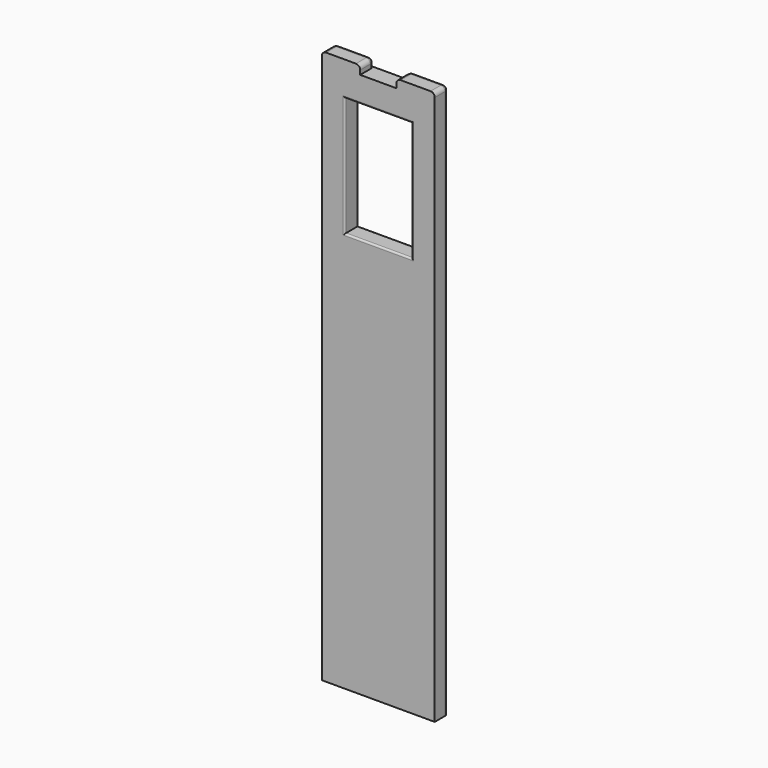
from build123d import *

# Parameters (mm, degrees)
F0_W     = 13.25
F0_H     = 65
F0_W_2   = 7.85
F0_H_2   = 14
F1_DEPTH = 2
F3_W     = 4.25
F3_H     = 2.1652186014
F4_DEPTH = 25
F5_R     = 0.5
F6_R     = 0.5
F7_R     = 0.2
F8_R     = 0.5


# Not quite as in the source:
# - the program builds the solid bodies; features that only make, move or delete a surface that nothing else refers to are left out


with BuildPart() as f1:
    # F0 (on Front) → F1 (new body)
    with BuildSketch(Plane.XZ):
        Rectangle(F0_W, F0_H)
        with Locations((0, 21.5)):
            Rectangle(F0_W_2, F0_H_2, mode=Mode.SUBTRACT)
    extrude(amount=F1_DEPTH)

    # F3 (on Front) → F4 (cut)
    with BuildSketch(Plane.XZ):
        with Locations((0, 32.5826093007)):
            Rectangle(F3_W, F3_H)
    extrude(amount=F4_DEPTH, mode=Mode.SUBTRACT)

    # F5
    f5_edges = [f1.edges().sort_by_distance(p)[0] for p in [
        (-2.125, -1, 32.5),
        (-6.625, -1, 32.5),
    ]]
    fillet(f5_edges, radius=F5_R)

    # F6
    f6_edges = [f1.edges().sort_by_distance(p)[0] for p in [
        (2.125, -1, 32.5),
        (6.625, -1, 32.5),
    ]]
    fillet(f6_edges, radius=F6_R)

    # F7
    f7_edges = [f1.edges().sort_by_distance(p)[0] for p in [
        (-3.925, -2, 21.5),
        (3.925, -2, 21.5),
        (3.925, 0, 21.5),
        (-3.925, 0, 21.5),
        (0, 0, 28.5),
        (0, -2, 28.5),
        (0, -2, 14.5),
        (0, 0, 14.5),
    ]]
    fillet(f7_edges, radius=F7_R)

    # F8
    f8_edges = [f1.edges().sort_by_distance(p)[0] for p in [
        (-6.625, 0, -0.25),
        (6.625, 0, -0.25),
    ]]
    fillet(f8_edges, radius=F8_R)


solid = f1.part
